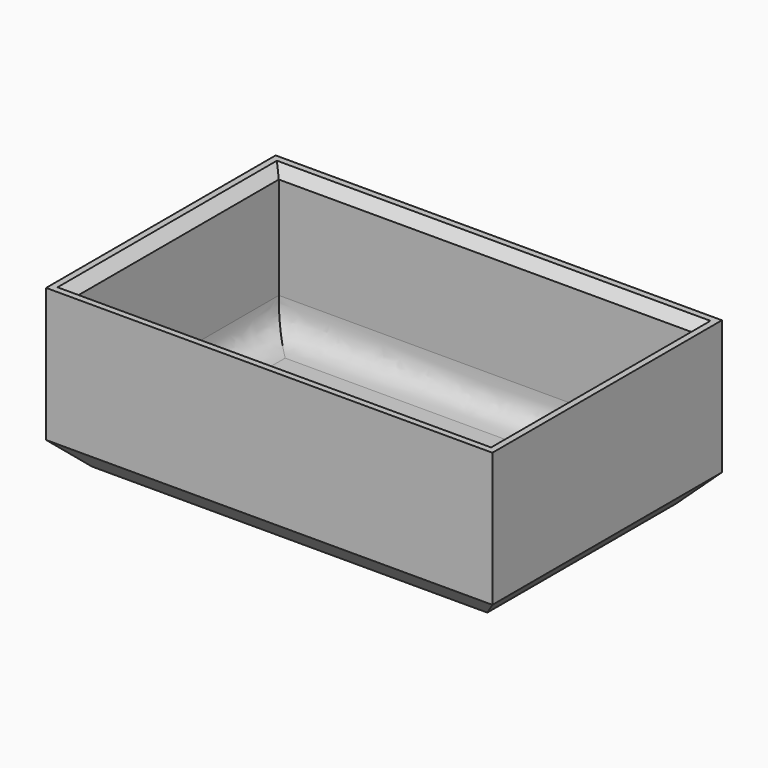
from build123d import *

# Parameters (mm, degrees)
F0_W        = 70
F0_H        = 45
F1_DEPTH    = 25
F2_T        = -2.5
F3_T1_DEPTH = 40
F3_T3_DEPTH = 65
F4_SIZE     = 4
F5_SIZE     = 1.5


# Not quite as in the source:
# - a fillet or chamfer that OpenCascade refuses, or shapes differently, is made with other operations: its cross-section is extruded or revolved along the edge and cut away or added


with BuildPart() as f1:
    # F0 (on Top) → F1 (new body)
    with BuildSketch(Plane.XY):
        with Locations((9.3095207959, -39.4999814034)):
            Rectangle(F0_W, F0_H)
    extrude(amount=F1_DEPTH)

    # F2
    f2_openings = [f1.faces().sort_by_distance(p)[0] for p in [
        (9.309521, -39.499981, 25),
    ]]
    offset(amount=F2_T, openings=f2_openings)

    # F3: fillet of radius 5 on 4 edges, made by hand

    # F3_s2 → F3_t1 (join)
    with BuildSketch(Plane.XZ.offset(19.4999814034)):
        with BuildLine():
            add(Edge.make_bspline(
                [(-23.1904792041, 7.5), (-23.1904792041, 2.5), (-18.1904792041, 2.5)],
                knots=[0, 0, 0, 1, 1, 1], degree=2, weights=[1, 1, 1]))
            Line((-18.1904792041, 2.5), (-23.1904792041, 2.5))
            Line((-23.1904792041, 2.5), (-23.1904792041, 7.5))
        make_face()
        with BuildLine():
            add(Edge.make_bspline(
                [(41.8095207959, 7.5), (41.8095207959, 2.5), (36.8095207959, 2.5)],
                knots=[0, 0, 0, 1, 1, 1], degree=2, weights=[1, 1, 1]))
            Line((36.8095207959, 2.5), (41.8095207959, 2.5))
            Line((41.8095207959, 2.5), (41.8095207959, 7.5))
        make_face()
    extrude(amount=F3_T1_DEPTH)

    # F3_s4 → F3_t3 (join)
    with BuildSketch(Plane.YZ.offset(-23.1904792041)):
        with BuildLine():
            add(Edge.make_bspline(
                [(-19.4999814034, 7.5), (-19.4999814034, 2.5), (-24.4999814034, 2.5)],
                knots=[0, 0, 0, 1, 1, 1], degree=2, weights=[1, 1, 1]))
            Line((-24.4999814034, 2.5), (-19.4999814034, 2.5))
            Line((-19.4999814034, 2.5), (-19.4999814034, 7.5))
        make_face()
        with BuildLine():
            add(Edge.make_bspline(
                [(-59.4999814034, 7.5), (-59.4999814034, 2.5), (-54.4999814034, 2.5)],
                knots=[0, 0, 0, 1, 1, 1], degree=2, weights=[1, 1, 1]))
            Line((-54.4999814034, 2.5), (-59.4999814034, 2.5))
            Line((-59.4999814034, 2.5), (-59.4999814034, 7.5))
        make_face()
    extrude(amount=F3_T3_DEPTH)

    # F4
    f4_edges = [f1.edges().sort_by_distance(p)[0] for p in [
        (9.309521, -61.999981, 0),
        (-25.690479, -39.499981, 0),
        (44.309521, -39.499981, 0),
        (9.309521, -16.999981, 0),
    ]]
    chamfer(f4_edges, length=F4_SIZE)

    # F5
    f5_edges = [f1.edges().sort_by_distance(p)[0] for p in [
        (9.309521, -19.499981, 25),
        (-23.190479, -39.499981, 25),
        (9.309521, -59.499981, 25),
        (41.809521, -39.499981, 25),
    ]]
    chamfer(f5_edges, length=F5_SIZE)


solid = f1.part
